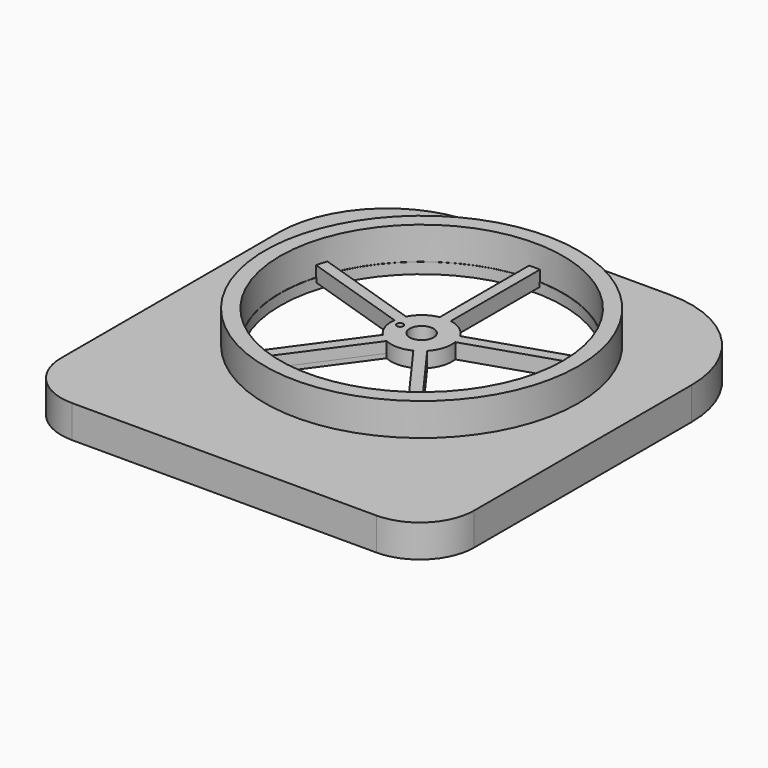
from build123d import *

# Parameters (mm, degrees)
F1_DEPTH  = 5
F3_DEPTH  = 10
F4_R      = 65
F5_DEPTH  = 25
F6_R      = 1.5
F6_R_2    = 5.5
F7_DEPTH  = 2
F8_R      = 5
F9_DEPTH  = 25
F10_R     = 1.5
F11_DEPTH = 25
F12_DEPTH = 25
F13_DEPTH = 25
F14_R     = 72.085840391
F14_R_2   = 65.1394362423
F15_DEPTH = 15
F16_DEPTH = 5


with BuildPart() as f1:
    # F0 (on Top) → F1 (new body)
    with BuildSketch(Plane.XY):
        with BuildLine():
            Line((139, 200), (49, 200))
            ThreePointArc((49, 200), (13.6446609407, 185.3553390593), (-1, 150))
            Line((-1, 150), (-1, 25))
            ThreePointArc((-1, 25), (6.3223304703, 7.3223304703), (24, 0))
            Line((24, 0), (164, 0))
            ThreePointArc((164, 0), (181.6776695297, 7.3223304703), (189, 25))
            Line((189, 25), (189, 150))
            ThreePointArc((189, 150), (174.3553390593, 185.3553390593), (139, 200))
        make_face()
    extrude(amount=F1_DEPTH)

    # F2 (on face) → F3 (join)
    with BuildSketch(Plane(origin=(0, 0, 0), x_dir=(1, 0, 0), z_dir=(0, 0, -1))):
        with BuildLine():
            Line((49, -200), (139, -200))
            ThreePointArc((139, -200), (174.3553390593, -185.3553390593), (189, -150))
            Line((189, -150), (189, -25))
            ThreePointArc((189, -25), (181.6776695297, -7.3223304703), (164, 0))
            Line((164, 0), (24, 0))
            ThreePointArc((24, 0), (6.3223304703, -7.3223304703), (-1, -25))
            Line((-1, -25), (-1, -150))
            ThreePointArc((-1, -150), (13.6446609407, -185.3553390593), (49, -200))
        make_face()
        with BuildLine():
            Line((186, -25), (186, -150))
            ThreePointArc((186, -150), (172.2340187158, -183.2340187158), (139, -197))
            Line((139, -197), (49, -197))
            ThreePointArc((49, -197), (15.7659812842, -183.2340187158), (2, -150))
            Line((2, -150), (2, -25))
            ThreePointArc((2, -25), (8.4436508139, -9.4436508139), (24, -3))
            Line((24, -3), (164, -3))
            ThreePointArc((164, -3), (179.5563491861, -9.4436508139), (186, -25))
        make_face(mode=Mode.SUBTRACT)
    extrude(amount=F3_DEPTH)

    # F4 (on face) → F5 (cut)
    with BuildSketch(Plane.XY.offset(5)):
        with Locations((94, 113.5067418218)):
            Circle(F4_R)
    extrude(amount=-F5_DEPTH, mode=Mode.SUBTRACT)

    # F8 (on face) → F9 (cut)
    with BuildSketch(Plane(origin=(0, 0, 3), x_dir=(1, 0, 0), z_dir=(0, 0, -1))):
        with Locations((94, -113.5067418218)):
            Circle(F8_R)
    extrude(amount=-F9_DEPTH, mode=Mode.SUBTRACT)

    # F10 (on face) → F11 (cut)
    with BuildSketch(Plane(origin=(0, 0, 3), x_dir=(1, 0, 0), z_dir=(0, 0, -1))):
        with Locations((94.0000067605, 105.5067418218)):
            Circle(F10_R)
        with Locations((86, 113.5067350613)):
            Circle(F10_R)
        with Locations((93.9999932395, 121.5067418218)):
            Circle(F10_R)
        with Locations((102, 113.5067485823)):
            Circle(F10_R)
    extrude(amount=-F11_DEPTH, mode=Mode.SUBTRACT)

    # F10 (on face) → F12 (cut)
    with BuildSketch(Plane(origin=(0, 0, 3), x_dir=(1, 0, 0), z_dir=(0, 0, -1))):
        with Locations((86, 113.5067350613)):
            Circle(F10_R)
        with Locations((94.0000067605, 105.5067418218)):
            Circle(F10_R)
        with Locations((102, 113.5067485823)):
            Circle(F10_R)
        with Locations((93.9999932395, 121.5067418218)):
            Circle(F10_R)
    extrude(amount=-F12_DEPTH, mode=Mode.SUBTRACT)

    # F8 (on face) → F13 (cut)
    with BuildSketch(Plane(origin=(0, 0, 3), x_dir=(1, 0, 0), z_dir=(0, 0, -1))):
        with Locations((94, -113.5067418218)):
            Circle(F8_R)
    extrude(amount=-F13_DEPTH, mode=Mode.SUBTRACT)


with BuildPart() as f7:
    # F6 (on face) → F7 (new body)
    with BuildSketch(Plane.XY.offset(5)):
        with BuildLine():
            Line((91.3489636779, 178.4526578321), (91.3489636779, 127.2534507522))
            ThreePointArc((91.3489636779, 127.2534507522), (85.6473138732, 124.7420715662), (81.5998298548, 120.005647912))
            Line((81.5998298548, 120.005647912), (32.947575311, 135.8137236794))
            ThreePointArc((32.947575311, 135.8137236794), (32.1347862264, 133.4490417079), (31.4135480954, 131.0548482151))
            Line((31.4135480954, 131.0548482151), (80.1068876178, 115.2334231289))
            ThreePointArc((80.1068876178, 115.2334231289), (80.7334444719, 109.0347730807), (83.9873097061, 103.7217516287))
            Line((83.9873097061, 103.7217516287), (53.9185627687, 62.3356719729))
            ThreePointArc((53.9185627687, 62.3356719729), (55.9163433267, 60.8319367021), (57.9704818098, 59.4061520007))
            Line((57.9704818098, 59.4061520007), (88.0646206604, 100.8271806269))
            ThreePointArc((88.0646206604, 100.8271806269), (94.1535038969, 99.5075833987), (100.2119872248, 100.9603792126))
            Line((100.2119872248, 100.9603792126), (130.2807341621, 59.5742995569))
            ThreePointArc((130.2807341621, 59.5742995569), (132.3282195336, 61.0096220209), (134.3189850648, 62.5226321076))
            Line((134.3189850648, 62.5226321076), (104.2248462142, 103.9436607337))
            ThreePointArc((104.2248462142, 103.9436607337), (107.3614261537, 109.3267548435), (107.8519095365, 115.5376534872))
            Line((107.8519095365, 115.5376534872), (156.5041640802, 131.3457292546))
            ThreePointArc((156.5041640803, 131.3457292546), (155.7717990733, 133.736542593), (154.9480213521, 136.0974189533))
            Line((154.9480213521, 136.0974189533), (106.2546818297, 120.2759938671))
            ThreePointArc((106.2546818297, 120.2759938671), (102.1043116043, 124.9225262197), (96.3489636779, 127.3082768683))
            Line((96.3489636779, 127.3082768683), (96.3489636779, 178.4642846451))
            ThreePointArc((96.3489636779, 178.4642846451), (93.8488518399, 178.5065660849), (91.3489636779, 178.4526578321))
        make_face()
        with Locations((84.0005032645, 113.607066474)):
            Circle(F6_R, mode=Mode.SUBTRACT)
        with Locations((94, 113.5067418218)):
            Circle(F6_R_2, mode=Mode.SUBTRACT)
    extrude(amount=-F7_DEPTH)



with BuildPart() as f15:
    # F14 (on face) → F15 (new body)
    with BuildSketch(Plane.XY.offset(5)):
        with Locations((94, 113.5067418218)):
            Circle(F14_R)
        with Locations((94, 113.5067418218)):
            Circle(F14_R_2, mode=Mode.SUBTRACT)
    extrude(amount=F15_DEPTH)


with BuildPart() as f7_1:
    add(f7.part)

    add(f15.part)  # F16 merges F15
    # F6 (on face) → F16 (join)
    with BuildSketch(Plane.XY.offset(5)):
        with BuildLine():
            Line((91.3489636779, 185.4482434715), (91.3489636779, 127.2534507522))
            ThreePointArc((91.3489636779, 127.2534507522), (85.6473138732, 124.7420715662), (81.5998298548, 120.005647912))
            Line((81.5998298548, 120.005647912), (26.3054357596, 137.9718856448))
            Line((26.3054357596, 137.9718856448), (24.7603507878, 133.2166030633))
            Line((24.7603507878, 133.2166030633), (80.1068876178, 115.2334231289))
            ThreePointArc((80.1068876178, 115.2334231289), (80.7334444719, 109.0347730807), (83.9873097061, 103.7217516287))
            Line((83.9873097061, 103.7217516287), (49.813494768, 56.6855305943))
            Line((49.813494768, 56.6855305943), (53.8585797398, 53.7466043329))
            Line((53.8585797398, 53.7466043329), (88.0646206604, 100.8271806269))
            ThreePointArc((88.0646206604, 100.8271806269), (94.1535038969, 99.5075833987), (100.2119872248, 100.9603792126))
            Line((100.2119872248, 100.9603792126), (134.3858021629, 53.9241581783))
            Line((134.3858021629, 53.9241581783), (138.4308871348, 56.8630844397))
            Line((138.4308871348, 56.8630844397), (104.2248462142, 103.9436607337))
            ThreePointArc((104.2248462142, 103.9436607337), (107.3614261537, 109.3267548435), (107.8519095365, 115.5376534872))
            Line((107.8519095365, 115.5376534872), (163.1463036316, 133.50389122))
            Line((163.1463036316, 133.50389122), (161.6012186598, 138.2591738015))
            Line((161.6012186598, 138.2591738015), (106.2546818297, 120.2759938671))
            ThreePointArc((106.2546818297, 120.2759938671), (102.1043116043, 124.9225262197), (96.3489636779, 127.3082768683))
            Line((96.3489636779, 127.3082768683), (96.3489636779, 185.4482434715))
            Line((96.3489636779, 185.4482434715), (91.3489636779, 185.4482434715))
        make_face()
        with Locations((84.0005032645, 113.607066474)):
            Circle(F6_R, mode=Mode.SUBTRACT)
        with Locations((94, 113.5067418218)):
            Circle(F6_R_2, mode=Mode.SUBTRACT)
    extrude(amount=F16_DEPTH)


solid = Compound([f1.part, f7_1.part])
